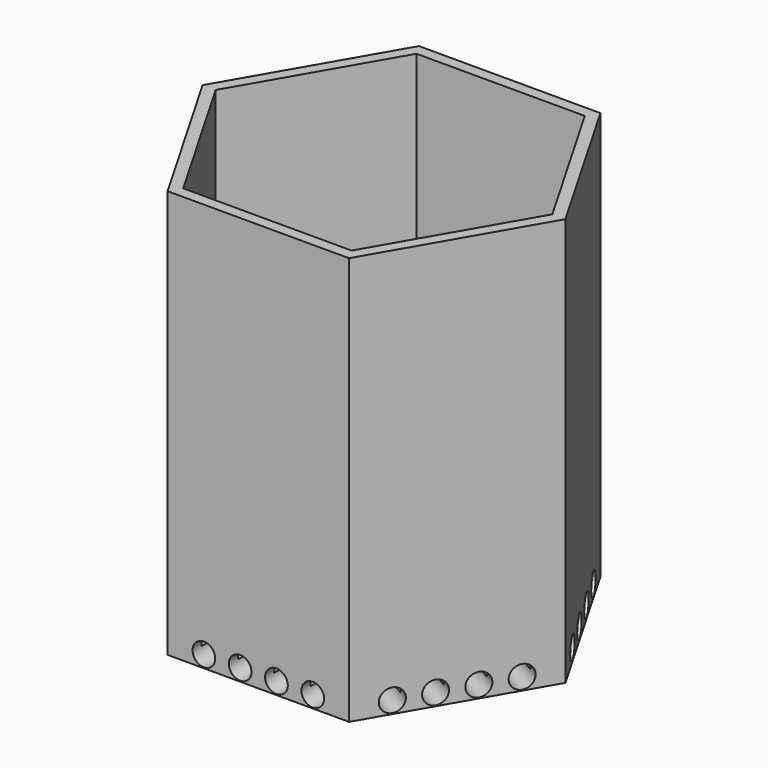
from build123d import *

# Parameters (mm, degrees)
F2_DEPTH = 228.6
F3_T     = -6.35
F4_R     = 6.35
F5_DEPTH = 203.2
F6_R     = 6.35
F7_DEPTH = 203.2
F8_R     = 6.35
F9_DEPTH = 203.2


with BuildPart() as f2:
    # F0 (on Top) → F2 (new body)
    with BuildSketch(Plane.XY):
        Polygon((-50.8, 87.9881810245), (-101.6, 0), (-50.8, -87.9881810245), (50.8, -87.9881810245), (101.6, 0), (50.8, 87.9881810245), align=None)
    extrude(amount=F2_DEPTH)

    # F3
    f3_openings = [f2.faces().sort_by_distance(p)[0] for p in [
        (0, 0, 228.6),
    ]]
    offset(amount=F3_T, openings=f3_openings)

    # F4 (on face) → F5 (cut)
    with BuildSketch(Plane(origin=(76.2, 43.9940905122, 0), x_dir=(-0.5, 0.8660254038, 0), z_dir=(0.8660254038, 0.5, 0))):
        with Locations((-30.48, 6.858)):
            Circle(F4_R)
        with Locations((-10.16, 6.858)):
            Circle(F4_R)
        with Locations((10.16, 6.858)):
            Circle(F4_R)
        with Locations((30.48, 6.858)):
            Circle(F4_R)
    extrude(amount=-F5_DEPTH, mode=Mode.SUBTRACT)

    # F6 (on face) → F7 (cut)
    with BuildSketch(Plane(origin=(-76.2, 43.9940905122, 0), x_dir=(-0.5, -0.8660254038, 0), z_dir=(-0.8660254038, 0.5, 0))):
        with Locations((-30.48, 6.858)):
            Circle(F6_R)
        with Locations((-10.16, 6.858)):
            Circle(F6_R)
        with Locations((10.16, 6.858)):
            Circle(F6_R)
        with Locations((30.48, 6.858)):
            Circle(F6_R)
    extrude(amount=-F7_DEPTH, mode=Mode.SUBTRACT)

    # F8 (on face) → F9 (cut)
    with BuildSketch(Plane(origin=(0, 87.9881810245, 0), x_dir=(-1, 0, 0), z_dir=(0, 1, 0))):
        with Locations((-30.48, 6.858)):
            Circle(F8_R)
        with Locations((-10.16, 6.858)):
            Circle(F8_R)
        with Locations((10.16, 6.858)):
            Circle(F8_R)
        with Locations((30.48, 6.858)):
            Circle(F8_R)
    extrude(amount=-F9_DEPTH, mode=Mode.SUBTRACT)


solid = f2.part
